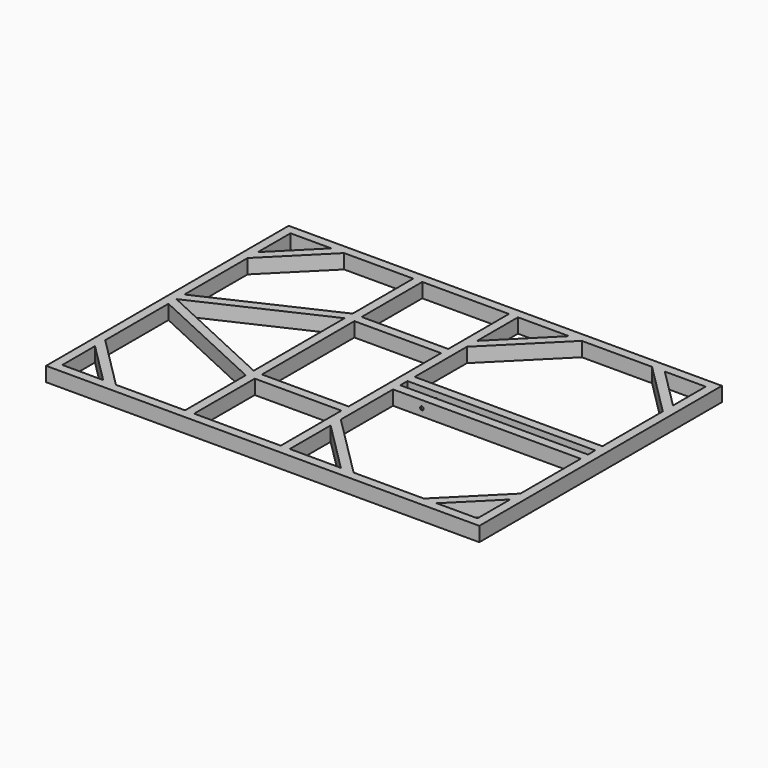
from build123d import *

# Parameters (mm, degrees)
F0_W     = 1524
F0_H     = 1066.8
F0_W_2   = 660.4
F0_H_2   = 31.75
F0_W_3   = 304.8
F1_DEPTH = 50.8
F3_R     = 6.35
F4_DEPTH = 127
F5_T     = -3.175


# Not quite as in the source:
# - a feature names something its author has since deleted; it is built from what else it names


with BuildPart() as f1:
    # F0 (on Top) → F1 (new body)
    with BuildSketch(Plane.XY):
        with Locations((762, -533.4)):
            Rectangle(F0_W, F0_H)
        Polygon((1011.4551224214, -1035.05), (831.85, -1035.05), (831.85, -855.4448775786), (831.85, -810.5435969733), (831.85, -581.025), (1492.25, -581.025), (1492.25, -788.03246), (1492.25, -832.48246), (1492.25, -846.4646214575), (1492.25, -891.3659020629), (1492.25, -1035.05), (1348.5659020629, -1035.05), (1303.6646214575, -1035.05), (1056.3564030267, -1035.05), align=None, mode=Mode.SUBTRACT)
        Polygon((31.75, -175.4340979371), (31.75, -31.75), (175.4340979371, -31.75), (220.3353785425, -31.75), (463.55, -31.75), (463.55, -298.45), (463.55, -333.4391527639), (463.55, -733.3608472361), (463.55, -768.35), (463.55, -1035.05), (220.3353785425, -1035.05), (175.4340979371, -1035.05), (31.75, -1035.05), (31.75, -891.3659020629), (31.75, -846.4646214575), (31.75, -832.48246), (31.75, -788.03246), (31.75, -568.3891527639), (31.75, -533.4), (31.75, -498.4108472361), (31.75, -220.3353785425), align=None, mode=Mode.SUBTRACT)
        Polygon((800.1, -1035.05), (495.3, -1035.05), (495.3, -768.35), (495.3, -736.6), (495.3, -330.2), (495.3, -298.45), (495.3, -31.75), (800.1, -31.75), (800.1, -298.45), (800.1, -330.2), (800.1, -736.6), (800.1, -768.35), align=None, mode=Mode.SUBTRACT)
        with Locations((1162.05, -533.4)):
            Rectangle(F0_W_2, F0_H_2, mode=Mode.SUBTRACT)
        Polygon((1348.5659020629, -31.75), (1492.25, -31.75), (1492.25, -175.4340979371), (1492.25, -220.3353785425), (1492.25, -485.775), (831.85, -485.775), (831.85, -256.2564030267), (831.85, -211.3551224214), (831.85, -31.75), (1011.4551224214, -31.75), (1056.3564030267, -31.75), (1303.6646214575, -31.75), align=None, mode=Mode.SUBTRACT)
        Polygon((463.55, -298.45), (31.75, -498.4108472361), (31.75, -533.4), (463.55, -333.4391527639), align=None)
        Polygon((463.55, -733.3608472361), (31.75, -533.4), (31.75, -568.3891527639), (463.55, -768.35), align=None)
        with Locations((647.7, -752.475)):
            Rectangle(F0_W_3, F0_H_2)
        with Locations((647.7, -314.325)):
            Rectangle(F0_W_3, F0_H_2)
        Polygon((831.85, -256.2564030267), (1056.3564030267, -31.75), (1011.4551224214, -31.75), (831.85, -211.3551224214), align=None)
        Polygon((831.85, -810.5435969733), (831.85, -855.4448775786), (1011.4551224214, -1035.05), (1056.3564030267, -1035.05), align=None)
        Polygon((220.3353785425, -31.75), (175.4340979371, -31.75), (31.75, -175.4340979371), (31.75, -220.3353785425), align=None)
        Polygon((220.3353785425, -1035.05), (31.75, -846.4646214575), (31.75, -891.3659020629), (175.4340979371, -1035.05), align=None)
        Polygon((1492.25, -846.4646214575), (1303.6646214575, -1035.05), (1348.5659020629, -1035.05), (1492.25, -891.3659020629), align=None)
        Polygon((1492.25, -220.3353785425), (1492.25, -175.4340979371), (1348.5659020629, -31.75), (1303.6646214575, -31.75), align=None)
    extrude(amount=F1_DEPTH)

    # F3 (on face) → F4 (cut)
    with BuildSketch(Plane(origin=(0, -485.775, 0), x_dir=(-1, 0, 0), z_dir=(0, 1, 0))):
        with Locations((-933.45, 25.4)):
            Circle(F3_R)
    extrude(amount=-F4_DEPTH, mode=Mode.SUBTRACT)

    # F5
    f5_openings = [f1.faces().sort_by_distance(p)[0] for p in [
        (939.8, -565.15, 25.4),
        (939.8, -501.65, 25.4),
    ]]
    offset(amount=F5_T, openings=f5_openings, kind=Kind.INTERSECTION)


solid = f1.part
